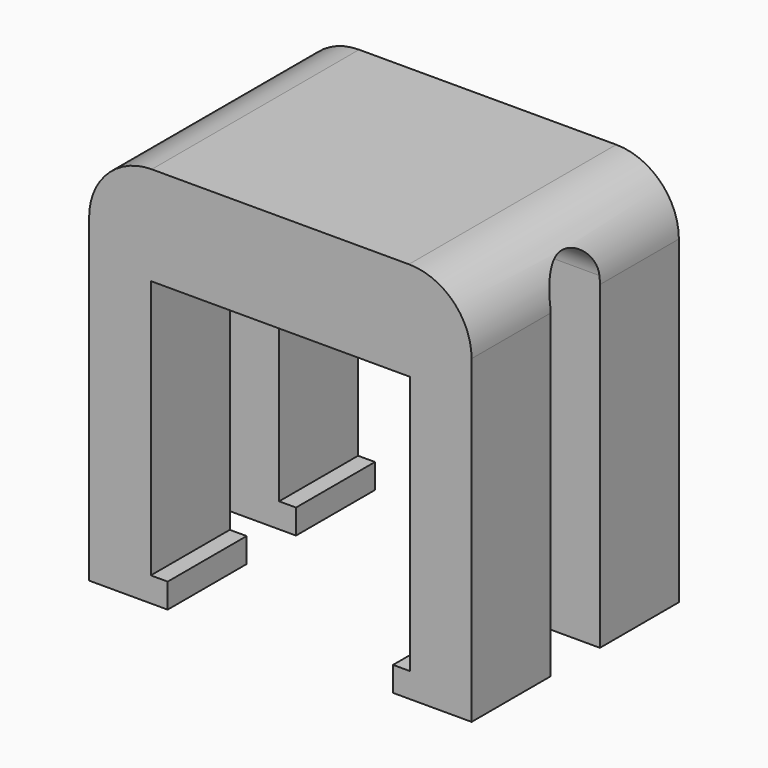
from build123d import *

# Parameters (mm, degrees)
F0_W         = 31
F0_H         = 21
F1_DEPTH     = 28
F2_W         = 21
F2_H         = 42
F3_DEPTH     = 50.8
F4_DEPTH     = 25.4
F6_DEPTH     = 25.4
F7_DEPTH     = 25.4
F8_DEPTH     = 2
F9_W         = 10.5
F9_H         = 2
F10_DEPTH    = 10.5
F11_DEPTH    = 10.5
F12_W        = 18.7637824565
F12_H        = 49.8975180089
F13_DEPTH    = 25.4
F14_DEPTH    = 25.4
F15_DEPTH    = 0.25
F16_DEPTH    = 0.25
F17_DEPTH    = 1
F18_T1_DEPTH = 46.4


# Not quite as in the source:
# - a fillet or chamfer that OpenCascade refuses, or shapes differently, is made with other operations: its cross-section is extruded or revolved along the edge and cut away or added


with BuildPart() as f1:
    # F0 (on Top) → F1 (new body)
    with BuildSketch(Plane.XY):
        Rectangle(F0_W, F0_H)
    extrude(amount=F1_DEPTH)

    # F2 (on Front) → F3 (cut)
    with BuildSketch(Plane.XZ):
        Rectangle(F2_W, F2_H)
    extrude(amount=-F3_DEPTH, mode=Mode.SUBTRACT)

    # F2 (on Front) → F4 (cut)
    with BuildSketch(Plane.XZ):
        Rectangle(F2_W, F2_H)
    extrude(amount=F4_DEPTH, mode=Mode.SUBTRACT)

    # F5 (on Right) → F6 (cut)
    with BuildSketch(Plane.YZ):
        with BuildLine():
            Line((0, 24.5501343161), (2.5, 24.5501343161))
            ThreePointArc((2.5, 24.5501343161), (0, 27.0501343161), (-2.5, 24.5501343161))
            Line((-2.5, 24.5501343161), (0, 24.5501343161))
        make_face()
        with BuildLine():
            Line((2.5, -28.5555105656), (2.5, 24.5501343161))
            ThreePointArc((2.5, 24.5501343161), (1.767766953, 22.7823673631), (0, 22.0501343161))
            Line((0, 22.0501343161), (0, -28.5555105656))
            Line((0, -28.5555105656), (2.5, -28.5555105656))
        make_face()
        with BuildLine():
            ThreePointArc((0, 22.0501343161), (1.767766953, 22.7823673631), (2.5, 24.5501343161))
            Line((2.5, 24.5501343161), (0, 24.5501343161))
            Line((0, 24.5501343161), (0, 22.0501343161))
        make_face()
        with BuildLine():
            Line((0, 24.5501343161), (-2.5, 24.5501343161))
            ThreePointArc((-2.5, 24.5501343161), (-1.767766953, 22.7823673631), (0, 22.0501343161))
            Line((0, 22.0501343161), (0, 24.5501343161))
        make_face()
        with BuildLine():
            ThreePointArc((0, 22.0501343161), (-1.767766953, 22.7823673631), (-2.5, 24.5501343161))
            Line((-2.5, 24.5501343161), (-2.5, -33.7370373309))
            Line((-2.5, -33.7370373309), (0, -33.7370373309))
            Line((0, -33.7370373309), (0, -28.5555105656))
            Line((0, -28.5555105656), (0, 22.0501343161))
        make_face()
    extrude(amount=-F6_DEPTH, mode=Mode.SUBTRACT)

    # F5 (on Right) → F7 (cut)
    with BuildSketch(Plane.YZ):
        with BuildLine():
            Line((0, 24.5501343161), (2.5, 24.5501343161))
            ThreePointArc((2.5, 24.5501343161), (0, 27.0501343161), (-2.5, 24.5501343161))
            Line((-2.5, 24.5501343161), (0, 24.5501343161))
        make_face()
        with BuildLine():
            Line((2.5, -28.5555105656), (2.5, 24.5501343161))
            ThreePointArc((2.5, 24.5501343161), (1.767766953, 22.7823673631), (0, 22.0501343161))
            Line((0, 22.0501343161), (0, -28.5555105656))
            Line((0, -28.5555105656), (2.5, -28.5555105656))
        make_face()
        with BuildLine():
            ThreePointArc((0, 22.0501343161), (1.767766953, 22.7823673631), (2.5, 24.5501343161))
            Line((2.5, 24.5501343161), (0, 24.5501343161))
            Line((0, 24.5501343161), (0, 22.0501343161))
        make_face()
        with BuildLine():
            Line((0, 24.5501343161), (-2.5, 24.5501343161))
            ThreePointArc((-2.5, 24.5501343161), (-1.767766953, 22.7823673631), (0, 22.0501343161))
            Line((0, 22.0501343161), (0, 24.5501343161))
        make_face()
        with BuildLine():
            ThreePointArc((0, 22.0501343161), (-1.767766953, 22.7823673631), (-2.5, 24.5501343161))
            Line((-2.5, 24.5501343161), (-2.5, -33.7370373309))
            Line((-2.5, -33.7370373309), (0, -33.7370373309))
            Line((0, -33.7370373309), (0, -28.5555105656))
            Line((0, -28.5555105656), (0, 22.0501343161))
        make_face()
    extrude(amount=F7_DEPTH, mode=Mode.SUBTRACT)

    # F8 (add): faces of the model
    f8_faces = [f1.faces().sort_by_distance(p)[0] for p in [
        (13, 6.5, 0),
        (13, -6.5, 0),
        (-13, -6.5, 0),
        (-13, 6.5, 0),
    ]]
    extrude(f8_faces, amount=F8_DEPTH)

    # F9 (on Right) → F10 (join)
    with BuildSketch(Plane.YZ):
        with Locations((-5.25, -1)):
            Rectangle(F9_W, F9_H)
        with Locations((5.25, -1)):
            Rectangle(F9_W, F9_H)
    extrude(amount=F10_DEPTH)

    # F11 (add): a face of the model
    f11_faces = [f1.faces().sort_by_distance(p)[0] for p in [
        (0, 0, -1),
    ]]
    extrude(f11_faces, amount=F11_DEPTH)

    # F12 (on Top) → F13 (cut)
    with BuildSketch(Plane.XY):
        Rectangle(F12_W, F12_H)
    extrude(amount=-F13_DEPTH, mode=Mode.SUBTRACT)

    # F14 (cut): a face of the model
    f14_faces = [f1.faces().sort_by_distance(p)[0] for p in [
        (10.5, 0, -1),
    ]]
    extrude(f14_faces, amount=-F14_DEPTH, mode=Mode.SUBTRACT)

    # F15 (add): faces of the model
    f15_faces = [f1.faces().sort_by_distance(p)[0] for p in [
        (9.3818912283, 6.5, -1),
        (9.3818912283, -6.5, -1),
    ]]
    extrude(f15_faces, amount=F15_DEPTH)

    # F16 (add): faces of the model
    f16_faces = [f1.faces().sort_by_distance(p)[0] for p in [
        (-9.3818912283, 6.5, -1),
        (-9.3818912283, -6.5, -1),
    ]]
    extrude(f16_faces, amount=F16_DEPTH)

    # F17 (add): a face of the model
    f17_faces = [f1.faces().sort_by_distance(p)[0] for p in [
        (0, 0, 28),
    ]]
    extrude(f17_faces, amount=F17_DEPTH)

    # F18: fillet of radius 5.08 on 2 edges, made by hand

    # F18_s2 → F18_t1 (cut)
    with BuildSketch(Plane.XZ.offset(-23.2)):
        with BuildLine():
            ThreePointArc((-15.5, 23.92), (-14.0121024484, 27.5121024484), (-10.42, 29))
            Line((-10.42, 29), (-15.5, 29))
            Line((-15.5, 29), (-15.5, 23.92))
        make_face()
        with BuildLine():
            ThreePointArc((15.5, 23.92), (14.0121024484, 27.5121024484), (10.42, 29))
            Line((10.42, 29), (15.5, 29))
            Line((15.5, 29), (15.5, 23.92))
        make_face()
    extrude(amount=F18_T1_DEPTH, mode=Mode.SUBTRACT)


solid = f1.part
